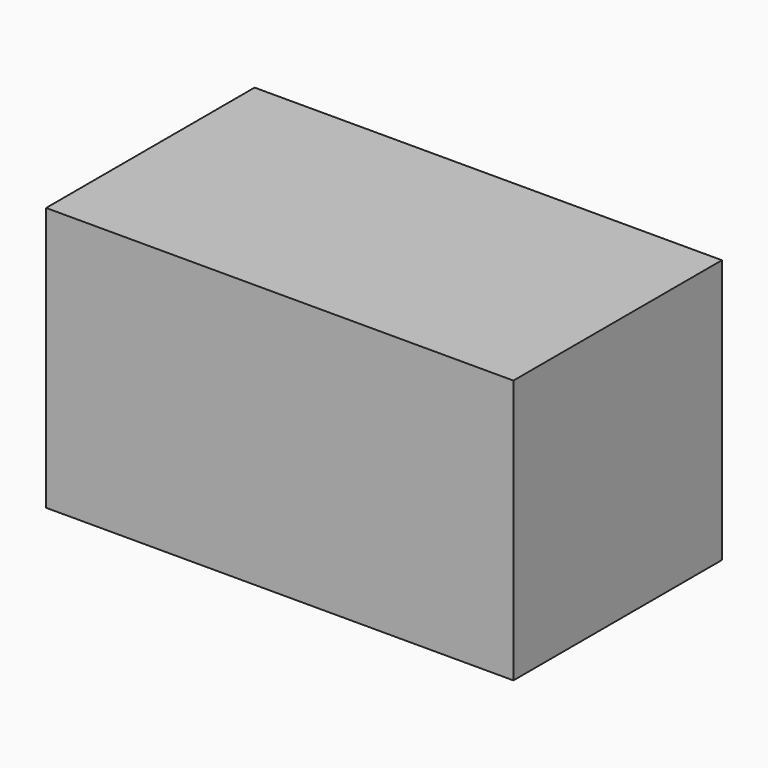
from build123d import *

# Parameters (mm, degrees)
F0_W     = 309.684753418
F0_H     = 174.9286130071
F1_DEPTH = 172.72


# Not quite as in the source:
# - the program builds the solid bodies; features that only make, move or delete a surface that nothing else refers to are left out


with BuildPart() as f1:
    # F0 (on Front) → F1 (new body)
    with BuildSketch(Plane.XZ):
        with Locations((0, -1.0427124798)):
            Rectangle(F0_W, F0_H)
    extrude(amount=F1_DEPTH)


solid = f1.part
